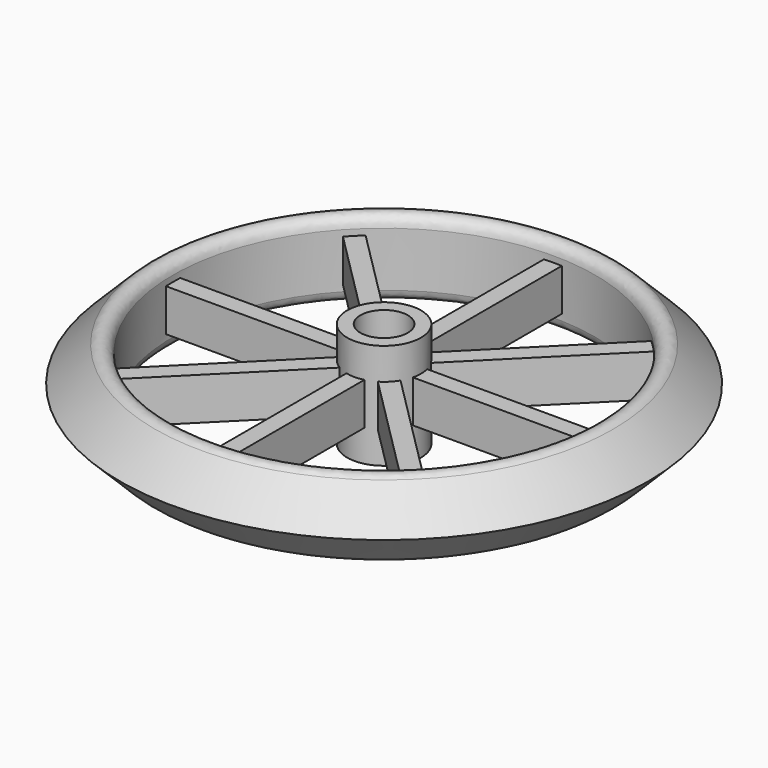
from build123d import *

# Parameters (mm, degrees)
F0_R     = 25
F1_DEPTH = 5
F2_SIZE  = 4.99999
F3_R     = 20.00001
F3_R_2   = 3.5
F4_DEPTH = 25
F3_R_3   = 2.25
F5_DEPTH = 12.5
F7_DEPTH = 2
F9_COUNT = 8
F10_R    = 1


# Not quite as in the source:
# - a fillet or chamfer is up to 0.001 mm smaller than in the source, because OpenCascade refuses the exact size


with BuildPart() as f1:
    # F0 (on Top) → F1 (new body, symmetric)
    with BuildSketch(Plane.XY):
        Circle(F0_R)
    extrude(amount=F1_DEPTH, both=True)

    # F2 (size 5 in the source; OpenCascade refuses exactly that, so slightly less here)
    f2_edges = [f1.edges().sort_by_distance(p)[0] for p in [
        (-25, 0, -5),
        (25, 0, 0),
        (-25, 0, 5),
    ]]
    chamfer(f2_edges, length=F2_SIZE)

    # F3 (on face) → F4 (cut)
    with BuildSketch(Plane.XY.offset(5)):
        Circle(F3_R)
        Circle(F3_R_2, mode=Mode.SUBTRACT)
    extrude(amount=-F4_DEPTH, mode=Mode.SUBTRACT)

    # F3 (on face) → F5 (cut, symmetric)
    with BuildSketch(Plane.XY.offset(5)):
        Circle(F3_R_3)
    extrude(amount=F5_DEPTH, both=True, mode=Mode.SUBTRACT)

    # F6 (on Top) → F7 (join, symmetric)
    with BuildSketch(Plane.XY):
        Polygon((0.8449734887, -2.9114803765), (0, -3.1155126635), (0, -21.5157922357), (0.8449734887, -21.5157922357), align=None)
        Polygon((0, -21.5157922357), (0, -3.1155126635), (-0.8449734887, -2.9114803765), (-0.8449734887, -21.5157922357), align=None)
    extrude(amount=F7_DEPTH, both=True)

    # F9: F1 ×8 about axis
    f9_axis = Axis((0, 0, 0.2882219851), (0, 0, -1))


with BuildPart() as f1_1:
    add(f1.part)
    for i in range(1, F9_COUNT):
        add(f1.part.rotate(f9_axis, i * 360 / F9_COUNT))

    # F10
    f10_edges = [f1_1.edges().sort_by_distance(p)[0] for p in [
        (-20.00001, 0, 5),
        (-20.00001, 0, -5),
    ]]
    fillet(f10_edges, radius=F10_R)


solid = f1_1.part
